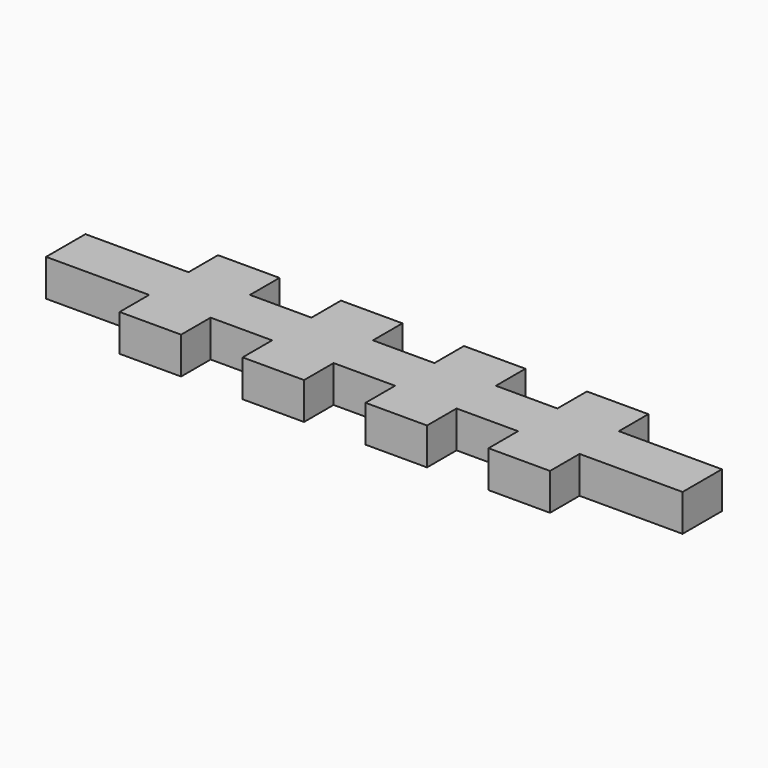
from build123d import *

# Parameters (mm, degrees)
F1_DEPTH = 7.62


# Not quite as in the source:
# - a feature names something its author has since deleted; it is built from what else it names


with BuildPart() as f1:
    # F0 (on Top) → F1 (new body)
    with BuildSketch(Plane.XY):
        Polygon((21.2852, -17.78), (21.2852, -25.4), (33.9852, -25.4), (33.9852, -17.78), (46.6852, -17.78), (46.6852, -25.4), (59.3852, -25.4), (59.3852, -17.78), (72.0852, -17.78), (72.0852, -25.4), (84.7852, -25.4), (84.7852, -17.78), (97.4852, -17.78), (97.4852, -25.4), (110.1852, -25.4), (110.1852, -17.78), (131.4704, -17.78), (131.4704, -7.62), (110.1852, -7.62), (110.1852, 0), (97.4852, 0), (97.4852, -7.62), (84.7852, -7.62), (84.7852, 0), (72.0852, 0), (72.0852, -7.62), (59.3852, -7.62), (59.3852, 0), (46.6852, 0), (46.6852, -7.62), (33.9852, -7.62), (33.9852, 0), (21.2852, 0), (21.2852, -7.62), (0, -7.62), (0, -17.78), align=None)
    extrude(amount=F1_DEPTH)


solid = f1.part
